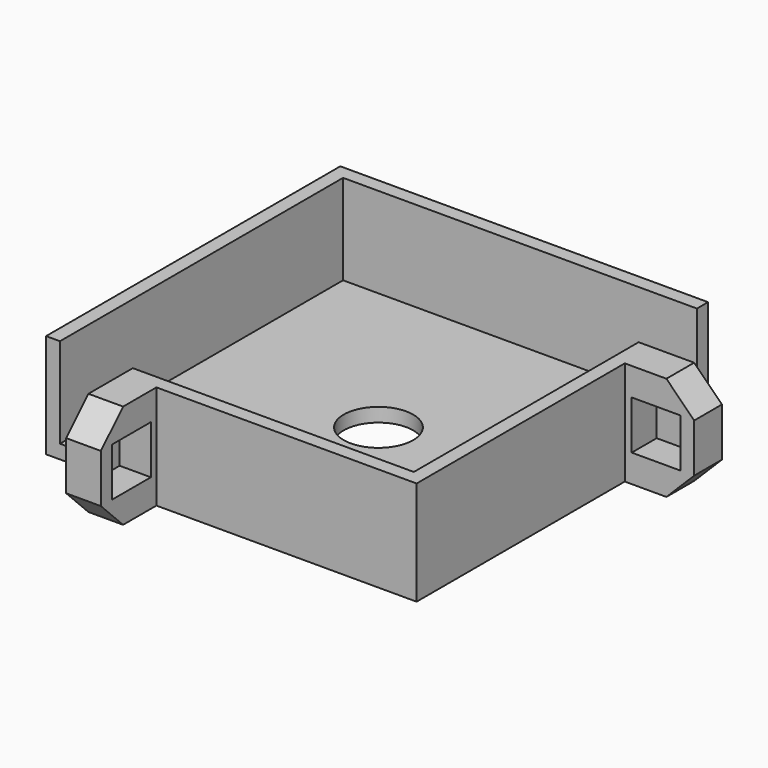
from build123d import *

# Parameters (mm, degrees)
F0_R      = 5
F1_DEPTH  = 2
F2_DEPTH  = 15
F3_W      = 5
F3_H      = 15
F4_DEPTH  = 10
F5_SIZE   = 4
F6_W      = 7
F6_H      = 7
F7_DEPTH  = 4.5
F8_W      = 5
F8_H      = 15
F9_DEPTH  = 10
F10_W     = 7
F10_H     = 7
F11_DEPTH = 4.5
F12_SIZE  = 4


with BuildPart() as f1:
    # F0 (on Top) → F1 (new body)
    with BuildSketch(Plane.XY):
        Polygon((25.5, 17.5), (25.5, 25.5), (-25.5, 25.5), (-25.5, -25.5), (-17.5, -25.5), (-15, -25.5), (25.5, -25.5), (25.5, 15), align=None)
        Circle(F0_R, mode=Mode.SUBTRACT)
    extrude(amount=F1_DEPTH)

    # F0 (on Top) → F2 (join)
    with BuildSketch(Plane.XY):
        Polygon((25.5, 27.5), (-27.5, 27.5), (-27.5, -25.5), (-25.5, -25.5), (-25.5, 25.5), (25.5, 25.5), align=None)
        Polygon((27.5, -27.5), (27.5, 15), (25.5, 15), (25.5, -25.5), (-15, -25.5), (-15, -27.5), align=None)
    extrude(amount=F2_DEPTH)

    # F3 (on face) → F4 (join)
    with BuildSketch(Plane.XZ.offset(27.5)):
        with Locations((-12.5, 7.5)):
            Rectangle(F3_W, F3_H)
    extrude(amount=F4_DEPTH)

    # F5
    f5_edges = [f1.edges().sort_by_distance(p)[0] for p in [
        (-12.5, -37.5, 15),
        (-12.5, -37.5, 0),
    ]]
    chamfer(f5_edges, length=F5_SIZE)

    # F6 (on face) → F7 (cut)
    with BuildSketch(Plane.YZ.offset(-10)):
        with Locations((-32, 7.5)):
            Rectangle(F6_W, F6_H)
    extrude(amount=-F7_DEPTH, mode=Mode.SUBTRACT)

    # F8 (on face) → F9 (join)
    with BuildSketch(Plane.YZ.offset(27.5)):
        with Locations((12.5, 7.5)):
            Rectangle(F8_W, F8_H)
    extrude(amount=F9_DEPTH)

    # F10 (on face) → F11 (cut)
    with BuildSketch(Plane.XZ.offset(-10)):
        with Locations((32, 7.5)):
            Rectangle(F10_W, F10_H)
    extrude(amount=-F11_DEPTH, mode=Mode.SUBTRACT)

    # F12
    f12_edges = [f1.edges().sort_by_distance(p)[0] for p in [
        (37.5, 12.5, 15),
        (37.5, 12.5, 0),
    ]]
    chamfer(f12_edges, length=F12_SIZE)


solid = f1.part
